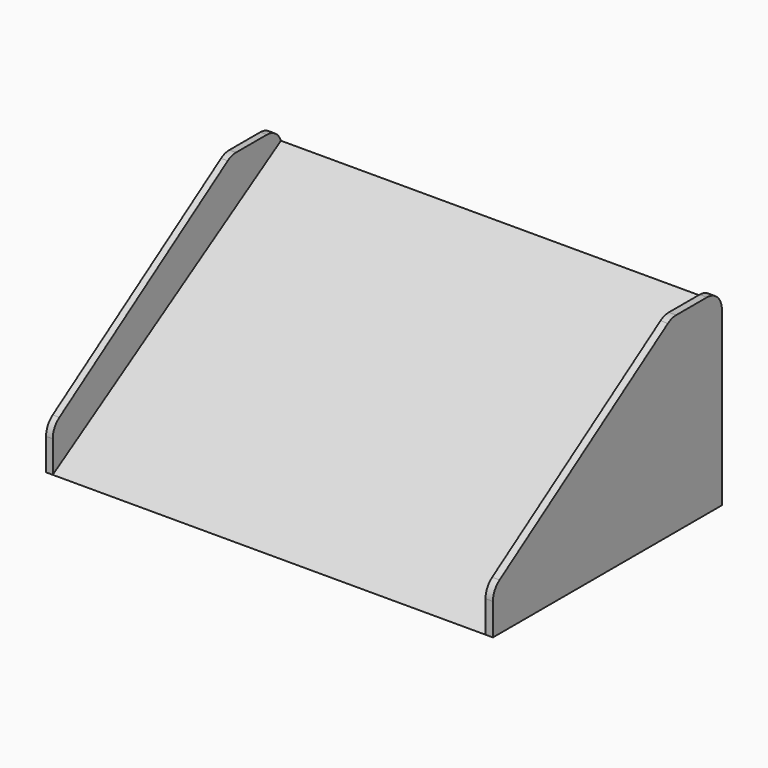
from build123d import *

# Parameters (mm, degrees)
F1_DEPTH    = 50
F2_T1_DEPTH = 529.8735996938
F0_R        = 2.5
F3_DEPTH    = 25
F0_W        = 1.7954435945
F0_H        = 76.8672563136
F0_W_2      = 1.9858591259
F4_DEPTH    = 51.2
F5_SIZE2    = 40
F5_SIZE     = 60
F5_2_SIZE2  = 40
F5_2_SIZE   = 60
F6_R        = 5


# Not quite as in the source:
# - a fillet or chamfer that OpenCascade refuses, or shapes differently, is made with other operations: its cross-section is extruded or revolved along the edge and cut away or added


with BuildPart() as f1:
    # F0 (on Top) → F1 (new body)
    with BuildSketch(Plane.XY):
        Polygon((-4.8924816283, 37.0864719152), (-57.8201711178, 37.0864719152), (-57.8201711178, -39.7807843983), (58.3985261619, -39.7807843983), (58.3985261619, 37.0864719152), (5.1028808584, 37.0864719152), align=None)
    extrude(amount=F1_DEPTH)

    # F2: chamfer of 80 x 50 on 1 edges, made by hand

    # F2_s2 → F2_t1 (cut)
    with BuildSketch(Plane.YZ.offset(-264.6476223249)):
        Polygon((40.2192156017, 50), (-39.7807843983, 0), (-39.7807843983, 50), align=None)
    extrude(amount=F2_T1_DEPTH, mode=Mode.SUBTRACT)

    # F0 (on Top) → F4 (join)
    with BuildSketch(Plane.XY):
        with Locations((-58.717892915, -1.3471562415)):
            Rectangle(F0_W, F0_H)
        with Locations((59.3914557248, -1.3471562415)):
            Rectangle(F0_W_2, F0_H)
    extrude(amount=F4_DEPTH)

    # F5
    f5_edges = [f1.edges().sort_by_distance(p)[0] for p in [
        (-58.717893, -39.780784, 51.2),
    ]]
    f5_side = f1.faces().sort_by_distance((-58.717893, -1.347156, 51.2))[0]
    chamfer(f5_edges, length=F5_SIZE, length2=F5_SIZE2, reference=f5_side)

    # F5#2
    f5_2_edges = [f1.edges().sort_by_distance(p)[0] for p in [
        (59.391456, -39.780784, 51.2),
    ]]
    f5_2_side = f1.faces().sort_by_distance((59.391456, -1.347156, 51.2))[0]
    chamfer(f5_2_edges, length=F5_2_SIZE, length2=F5_2_SIZE2, reference=f5_2_side)

    # F6
    f6_edges = [f1.edges().sort_by_distance(p)[0] for p in [
        (59.391456, 37.086472, 51.2),
        (59.391456, 20.219216, 51.2),
        (-58.717893, 20.219216, 51.2),
        (59.391456, -39.780784, 11.2),
        (-58.717893, -39.780784, 11.2),
    ]]
    fillet(f6_edges, radius=F6_R)


with BuildPart() as f3:
    # F0 (on Top) → F3 (new body)
    with BuildSketch(Plane.XY):
        with BuildLine():
            ThreePointArc((5.1028808584, 42.6884462108), (-0.0001560601, 47.4719877743), (-4.8924816283, 42.4731472871))
            ThreePointArc((-4.8924816283, 42.4731472871), (-0.0001560601, 37.4743067999), (5.1028808584, 42.2578483634))
            Line((5.1028808584, 42.2578483634), (5.1028808584, 42.6884462108))
        make_face()
        with Locations((0.1075183717, 42.4731472871)):
            Circle(F0_R, mode=Mode.SUBTRACT)
        with BuildLine():
            Line((-4.8924816283, 42.4731472871), (-4.8924816283, 37.0864719152))
            Line((-4.8924816283, 37.0864719152), (5.1028808584, 37.0864719152))
            Line((5.1028808584, 37.0864719152), (5.1028808584, 42.2578483634))
            ThreePointArc((5.1028808584, 42.2578483634), (-0.0001560601, 37.4743067999), (-4.8924816283, 42.4731472871))
        make_face()
    extrude(amount=F3_DEPTH)


solid = Compound([f1.part, f3.part])
